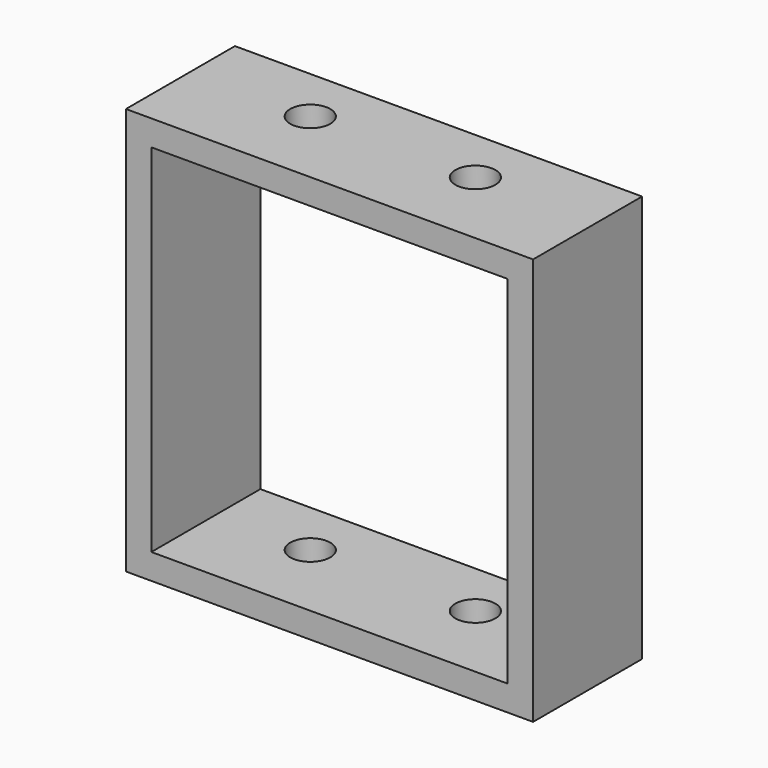
from build123d import *

# Parameters (mm, degrees)
F0_W          = 50.8
F0_H          = 50.8
F0_W_2        = 44.45
F0_H_2        = 44.45
F1_DEPTH      = 10
F1_DEPTH_BACK = 7
F3_D          = 5
F3_DEPTH      = 25.401
F4_D          = 5


# Not quite as in the source:
# - a feature names something its author has since deleted; it is built from what else it names


with BuildPart() as f1:
    # F0 (on Front) → F1 (new body, two sides)
    with BuildSketch(Plane.XZ) as f1_sk:
        Rectangle(F0_W, F0_H)
        Rectangle(F0_W_2, F0_H_2, mode=Mode.SUBTRACT)
    extrude(amount=F1_DEPTH)
    extrude(f1_sk.sketch, amount=-F1_DEPTH_BACK)

    # F3 (through all, one way)
    with BuildSketch(Plane(origin=(0, 0, 0), x_dir=(1, 0, 0), z_dir=(0, 0, -1))):
        with Locations((-10.4, 0), (10.2, 0)):
            Circle(F3_D / 2)
    extrude(amount=-F3_DEPTH, mode=Mode.SUBTRACT)

    # F4 (through all)
    with Locations(Plane.XY):
        with Locations((-10.4, 0), (10.2, 0)):
            Hole(F4_D / 2)


solid = f1.part
